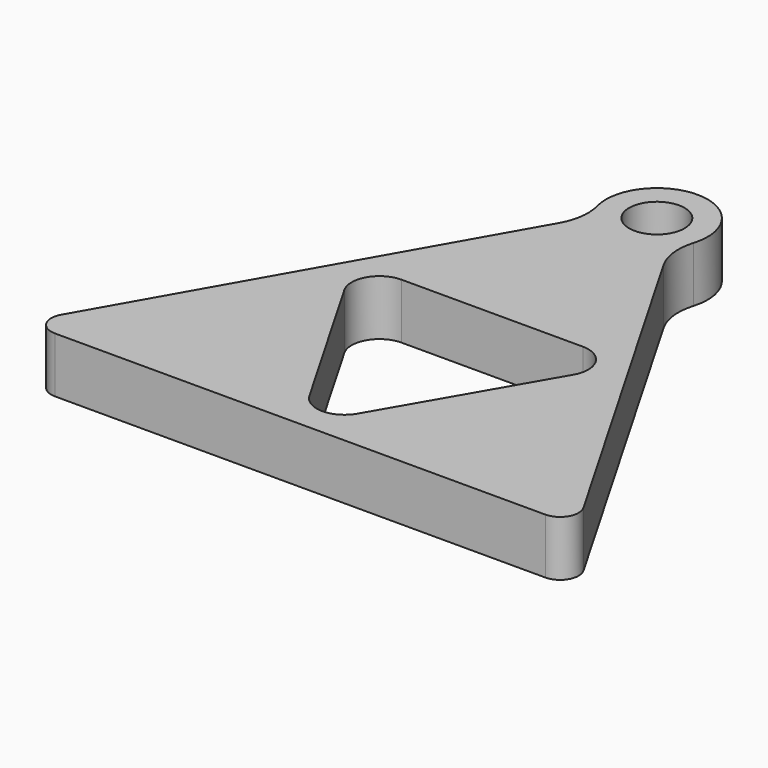
from build123d import *

# Parameters (mm, degrees)
F0_R     = 1.5
F1_DEPTH = 3
F2_R     = 3


# Not quite as in the source:
# - a feature names something its author has since deleted; it is built from what else it names


with BuildPart() as f1:
    # F0 (on Top) → F1 (new body)
    with BuildSketch(Plane.XY):
        with BuildLine():
            ThreePointArc((-14.1339745962, -7.1602540378), (-14.1339745962, -8.1602540378), (-13.2679491924, -8.6602540378))
            Line((-13.2679491924, -8.6602540378), (13.2679491924, -8.6602540378))
            ThreePointArc((13.2679491924, -8.6602540378), (14.1339745962, -8.1602540378), (14.1339745962, -7.1602540378))
            Line((14.1339745962, -7.1602540378), (2.096494358, 13.6892733298))
            ThreePointArc((2.096494358, 13.6892733298), (0.0937033826, 18.2173425378), (-2.2128362603, 13.8361945924))
            Line((-2.2128362603, 13.8361945924), (-14.1339745962, -7.1602540378))
        make_face()
        with BuildLine():
            Line((-4.9019237886, 4.3301270189), (4.9019237886, 4.3301270189))
            ThreePointArc((4.9019237886, 4.3301270189), (6.2009618943, 3.5801270189), (6.2009618943, 2.0801270189))
            Line((6.2009618943, 2.0801270189), (1.2990381057, -6.4102540378))
            ThreePointArc((1.2990381057, -6.4102540378), (0, -7.1602540378), (-1.2990381057, -6.4102540378))
            Line((-1.2990381057, -6.4102540378), (-6.2009618943, 2.0801270189))
            ThreePointArc((-6.2009618943, 2.0801270189), (-6.2009618943, 3.5801270189), (-4.9019237886, 4.3301270189))
        make_face(mode=Mode.SUBTRACT)
        with Locations((0, 15.468939424)):
            Circle(F0_R, mode=Mode.SUBTRACT)
    extrude(amount=F1_DEPTH)

    # F2
    f2_edges = [f1.edges().sort_by_distance(p)[0] for p in [
        (-2.212836, 13.836195, 1.5),
        (2.096494, 13.689273, 1.5),
    ]]
    fillet(f2_edges, radius=F2_R)


solid = f1.part
